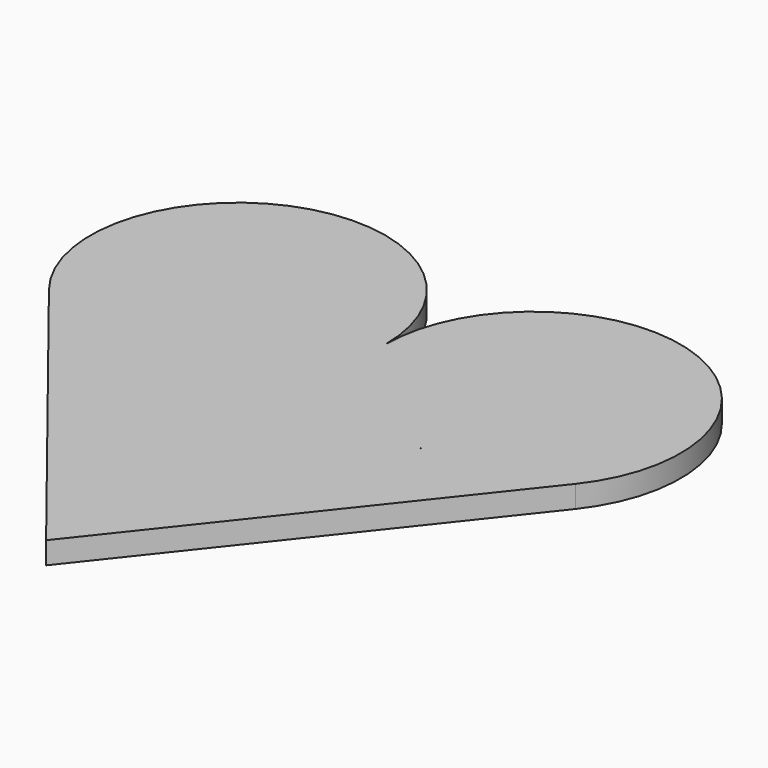
from build123d import *

# Parameters (mm, degrees)
F1_DEPTH = 6
F2_DEPTH = 4
F3_DEPTH = 2


with BuildPart() as f1:
    # F0 (on Top) → F1 (new body)
    with BuildSketch(Plane.XY):
        with BuildLine():
            Line((0, -75), (71.3659359191, 15.1770657673))
            ThreePointArc((71.3659359191, 15.1770657673), (53.1408249977, 77.7798718682), (0, 40))
            ThreePointArc((0, 40), (-53.1408249977, 77.7798718682), (-71.3659359191, 15.1770657673))
            Line((-71.3659359191, 15.1770657673), (0, -75))
        make_face()
        with BuildLine():
            ThreePointArc((-62.3608017817, 13.1737193764), (-46.5622648655, 68.0350424728), (0, 35))
            ThreePointArc((0, 35), (46.5622648655, 68.0350424728), (62.3608017817, 13.1737193764))
            Line((62.3608017817, 13.1737193764), (35, -21.125))
            Line((35, -21.125), (23.9316239316, -35))
            Line((23.9316239316, -35), (0, -65))
            Line((0, -65), (-62.3608017817, 13.1737193764))
        make_face(mode=Mode.SUBTRACT)
    extrude(amount=-F1_DEPTH)

    # F0 (on Top) → F2 (join)
    with BuildSketch(Plane.XY):
        with BuildLine():
            ThreePointArc((62.3608017817, 13.1737193764), (46.5622648655, 68.0350424728), (0, 35))
            ThreePointArc((0, 35), (-46.5622648655, 68.0350424728), (-62.3608017817, 13.1737193764))
            Line((-62.3608017817, 13.1737193764), (0, -65))
            Line((0, -65), (23.9316239316, -35))
            Line((23.9316239316, -35), (35, -21.125))
            Line((35, -21.125), (62.3608017817, 13.1737193764))
        make_face()
        with BuildLine():
            Line((35, 6.6666666667), (0, -40))
            Line((0, -40), (-36, 8))
            ThreePointArc((-36, 8), (-26.3245553203, 38.973665961), (0, 20))
            ThreePointArc((0, 20), (26.3245553203, 38.973665961), (36, 8))
            Line((36, 8), (35, 6.6666666667))
        make_face(mode=Mode.SUBTRACT)
    extrude(amount=-F2_DEPTH)

    # F0 (on Top) → F3 (join)
    with BuildSketch(Plane.XY):
        with BuildLine():
            Line((-36, 8), (0, -40))
            Line((0, -40), (35, 6.6666666667))
            Line((35, 6.6666666667), (35, 6.7712434447))
            ThreePointArc((35, 6.7712434447), (35.5121713718, 7.3757162844), (36, 8))
            ThreePointArc((36, 8), (26.3245553203, 38.973665961), (0, 20))
            ThreePointArc((0, 20), (-26.3245553203, 38.973665961), (-36, 8))
        make_face()
    extrude(amount=-F3_DEPTH)


solid = f1.part
